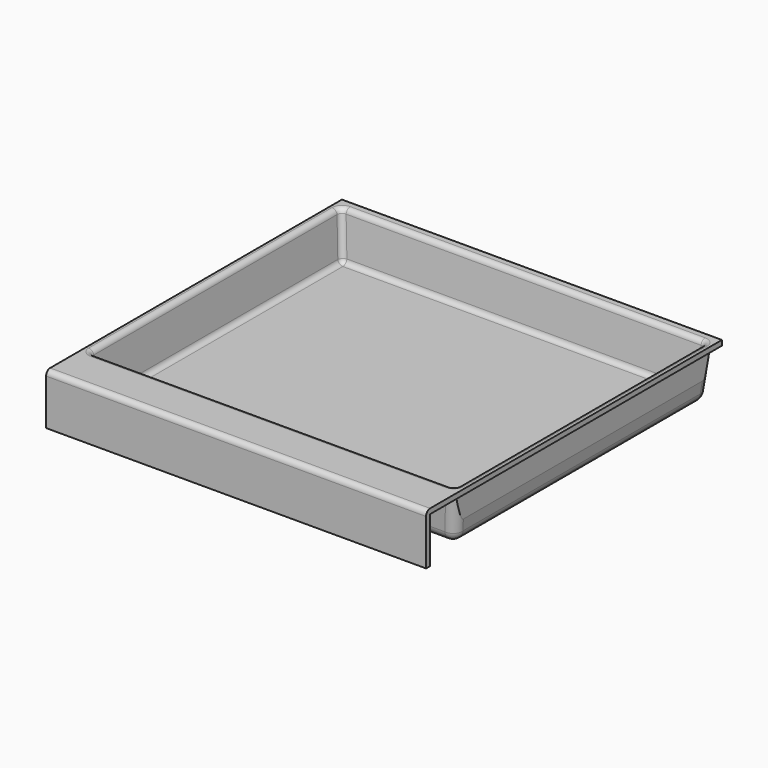
from build123d import *

# Parameters (mm, degrees)
F0_W                   = 949.325
F0_H                   = 923.925
F1_DEPTH               = 127
F2_W                   = 914.4
F2_H                   = 787.4
F3_DEPTH               = 114.3
DRAFT_F3_DRAFTED_ANGLE = 6
F4_R                   = 12.7
F6_T                   = 12.7
F7_W                   = 911.225
F7_H                   = 114.3
F8_DEPTH               = 12.7
F9_W                   = 936.625
F9_H                   = 114.3
F10_DEPTH              = 12.7
F11_W                  = 898.525
F11_H                  = 114.3
F12_DEPTH              = 12.7


# Not quite as in the source:
# - two fillets or chamfers of one size are made in one step
# - an extrude with a draft is written as a straight extrude whose walls are then drafted
# - a shell that OpenCascade refuses in one call is made with other operations: the cavity is built on its own and cut out


with BuildPart() as f1:
    # F0 (on Top) → F1 (new body)
    with BuildSketch(Plane.XY):
        with Locations((474.6625, -461.9625)):
            Rectangle(F0_W, F0_H)
    extrude(amount=F1_DEPTH)


with BuildPart() as f3_drafted:
    # F2 (on face) → F3 (new body)
    with BuildSketch(Plane.XY.offset(127)):
        with Locations((474.6625, -418.524437584)):
            Rectangle(F2_W, F2_H)
    extrude(amount=-F3_DEPTH)

    # draft_F3_drafted
    draft_f3_drafted_walls = [f3_drafted.faces().sort_by_distance(p)[0] for p in [
        (17.4625, -418.524437584, 50.8),
        (474.6625, -812.224437584, 50.8),
        (931.8625, -418.524437584, 50.8),
        (474.6625, -24.824437584, 50.8),
    ]]
    draft(draft_f3_drafted_walls, neutral_plane=Plane(origin=(0, 0, 127), x_dir=(1, 0, 0), z_dir=(0, 0, -1)), angle=DRAFT_F3_DRAFTED_ANGLE)


with BuildPart() as f1_1:
    add(f1.part)

    # join_F3_drafted: cut F3_drafted
    add(f3_drafted.part, mode=Mode.SUBTRACT)

    # F4
    f4_edges = [f1_1.edges().sort_by_distance(p)[0] for p in [
        (17.4625, -418.524438, 127),
        (474.6625, -812.224438, 127),
        (474.6625, -24.824438, 127),
        (474.6625, -923.925, 127),
        (931.8625, -418.524438, 127),
        (23.469207, -30.831145, 69.85),
        (23.469207, -806.217731, 69.85),
        (29.475914, -418.524438, 12.7),
        (925.855793, -806.217731, 69.85),
        (474.6625, -800.211023, 12.7),
        (925.855793, -30.831145, 69.85),
        (919.849086, -418.524438, 12.7),
        (474.6625, -36.837852, 12.7),
    ]]
    fillet(f4_edges, radius=F4_R)

    # F6: shell of thickness 12.7, made by hand


with BuildPart() as f6_core1:
    # F6_t2: copy of F1
    add(f1_1.part)

    # the walls: a layer under each face that stays
    f6_faces = [f6_core1.faces().sort_by_distance(p)[0] for p in [
        (949.325, -461.9625, 63.5),
        (474.6625, -923.925, 57.15),
        (67.8089285714, -846.1375, 127),
        (474.6625, 0, 63.5),
        (0, -461.9625, 63.5),
        (19.2740919361, -26.6360295201, 123.9177852818),
        (19.2740919361, -810.4128456479, 123.9177852818),
        (930.0509080639, -26.6360295201, 123.9177852818),
        (930.0509080639, -810.4128456479, 123.9177852818),
        (23.4692070454, -418.524437584, 69.85),
        (27.1532640456, -34.5152016296, 69.916410387),
        (27.1532640456, -802.5336735384, 69.916410387),
        (474.6625, -30.8311446294, 69.85),
        (474.6625, -806.2177305385, 69.85),
        (922.1717359544, -34.5152016296, 69.916410387),
        (922.1717359544, -802.5336735384, 69.916410387),
        (925.8557929546, -418.524437584, 69.85),
        (32.4130867527, -418.524437584, 15.9620607164),
        (34.9020812299, -42.2640188139, 15.9620607164),
        (34.9020812299, -794.7848563541, 15.9620607164),
        (474.6625, -39.7750243367, 15.9620607164),
        (474.6625, -797.2738508313, 15.9620607164),
        (914.4229187701, -42.2640188139, 15.9620607164),
        (914.4229187701, -794.7848563541, 15.9620607164),
        (916.9119132473, -418.524437584, 15.9620607164),
        (474.6625, -418.524437584, 12.7),
    ]]
    thicken(f6_faces, amount=-F6_T, mode=Mode.SUBTRACT)


with BuildPart() as f1_2:
    add(f1_1.part)

    # what is left inside the walls is the cavity
    f6_cavity = [f6_core1.part.solids().sort_by_distance(p)[0] for p in [
        (705.64375, -811.388889, 0.127),
    ]]
    add(f6_cavity, mode=Mode.SUBTRACT)

    # F7 (on face) → F8 (cut)
    with BuildSketch(Plane.YZ.offset(949.325)):
        with Locations((-455.6125, 57.15)):
            Rectangle(F7_W, F7_H)
    extrude(amount=-F8_DEPTH, mode=Mode.SUBTRACT)

    # F9 (on face) → F10 (cut)
    with BuildSketch(Plane(origin=(0, 0, 0), x_dir=(-1, 0, 0), z_dir=(0, 1, 0))):
        with Locations((-468.3125, 57.15)):
            Rectangle(F9_W, F9_H)
    extrude(amount=-F10_DEPTH, mode=Mode.SUBTRACT)

    # F11 (on face) → F12 (cut)
    with BuildSketch(Plane(origin=(0, 0, 0), x_dir=(0, -1, 0), z_dir=(-1, 0, 0))):
        with Locations((461.9625, 57.15)):
            Rectangle(F11_W, F11_H)
    extrude(amount=-F12_DEPTH, mode=Mode.SUBTRACT)


solid = f1_2.part
